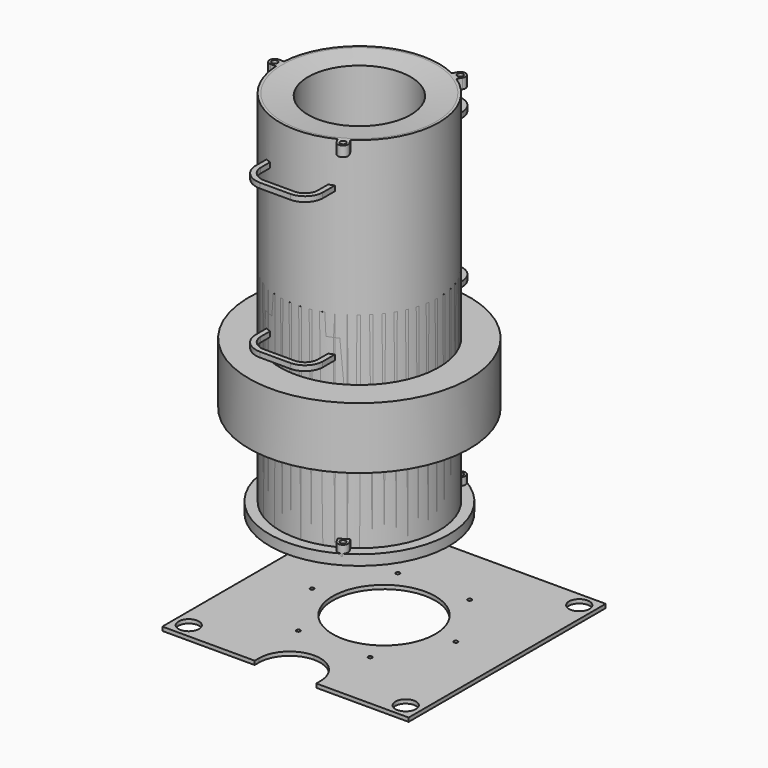
from build123d import *

# Parameters (mm, degrees)
F0_R      = 25.4
F0_R_2    = 4.7625
F1_DEPTH  = 9.525
F2_R      = 3.175
F3_DEPTH  = 12.7
F7_START  = -488.95
F6_R      = 7.14375
F7_DEPTH  = 25.4
F8_START  = -88.9
F8_DEPTH  = 12.7
F4_W      = 6.35
F4_H      = 381
F10_START = 266.7
F10_DEPTH = 12.7
F11_START = 355.6
F11_DEPTH = 25.4


# Not quite as in the source:
# - a feature names something its author has since deleted; it is built from what else it names


with BuildPart() as f1:
    # F0 (on Top) → F1 (new body)
    with BuildSketch(Plane.XY):
        with BuildLine():
            Line((609.6, 0), (0, 0))
            Line((0, 0), (0, -609.6))
            Line((0, -609.6), (228.6, -609.6))
            Line((228.6, -609.6), (228.6, -596.9))
            ThreePointArc((228.6, -596.9), (250.9184632736, -543.0184632736), (304.8, -520.7))
            ThreePointArc((304.8, -520.7), (358.6815367264, -543.0184632736), (381, -596.9))
            Line((381, -596.9), (381, -609.6))
            Line((381, -609.6), (609.6, -609.6))
            Line((609.6, -609.6), (609.6, 0))
        make_face()
        with Locations((36.3869200975, -573.2130799025)):
            Circle(F0_R, mode=Mode.SUBTRACT)
        with Locations((215.9, -458.7793167929)):
            Circle(F0_R_2, mode=Mode.SUBTRACT)
        with BuildLine():
            ThreePointArc((398.4625, -458.7793167929), (391.31875, -462.9037627784), (391.31875, -454.6548708073))
            ThreePointArc((391.31875, -454.6548708073), (396.08125, -454.6548708073), (398.4625, -458.7793167929))
        make_face(mode=Mode.SUBTRACT)
        with Locations((573.2130799025, -573.2130799025)):
            Circle(F0_R, mode=Mode.SUBTRACT)
        with Locations((127, -304.8)):
            Circle(F0_R_2, mode=Mode.SUBTRACT)
        with Locations((36.3869200975, -36.3869200975)):
            Circle(F0_R, mode=Mode.SUBTRACT)
        with Locations((215.9, -150.8206832071)):
            Circle(F0_R_2, mode=Mode.SUBTRACT)
        with BuildLine():
            ThreePointArc((368.3, -414.7852262806), (337.670018728, -427.4725799387), (304.8, -431.8))
            ThreePointArc((304.8, -431.8), (214.9974387893, -214.9974387893), (431.8, -304.8))
            ThreePointArc((431.8, -304.8), (414.7852262806, -368.3), (368.3, -414.7852262806))
        make_face(mode=Mode.SUBTRACT)
        with Locations((482.6, -304.8)):
            Circle(F0_R_2, mode=Mode.SUBTRACT)
        with Locations((393.7, -150.8206832071)):
            Circle(F0_R_2, mode=Mode.SUBTRACT)
        with Locations((573.2130799025, -36.3869200975)):
            Circle(F0_R, mode=Mode.SUBTRACT)
    extrude(amount=-F1_DEPTH)


with BuildPart() as f3:
    # F2 (on Top) → F3 (new body)
    with BuildSketch(Plane.XY):
        with BuildLine():
            ThreePointArc((13.051756509, -139.0889702745), (103.2942892524, -94.0551955388), (139.7, 0))
            ThreePointArc((139.7, 0), (93.8175544432, 103.5101757234), (-13.6909302547, 139.0275096115))
            Line((-13.6909302547, 139.0275096115), (-12.1714498273, 123.2253371732))
            ThreePointArc((-12.1714498273, 123.2253371732), (-9.8348553071, 122.5039217735), (-8.7041161086, 120.3356175983))
            ThreePointArc((-8.7041161086, 120.3356175983), (3.9055898005, 120.5867690433), (16.4726167188, 119.5201882463))
            ThreePointArc((16.4726167188, 119.5201882463), (19.8499978481, 122.2114111712), (22.7869087337, 119.0453507527))
            ThreePointArc((22.7869087337, 119.0453507527), (22.7745623185, 118.7656235596), (22.7376190943, 118.4880718804))
            ThreePointArc((22.7376190943, 118.4880718804), (34.982662471, 115.467033505), (46.8454269076, 111.1842096605))
            ThreePointArc((46.8454269076, 111.1842096606), (50.4041591942, 113.0209407678), (52.9298531544, 109.9130433005))
            ThreePointArc((52.9298531544, 109.9130433005), (52.853938074, 109.2229000827), (52.6298231316, 108.5657598745))
            ThreePointArc((52.6298231316, 108.5657598745), (63.6757245056, 102.4784104516), (74.0257986684, 95.271210927))
            ThreePointArc((74.0257986684, 95.271210927), (77.5564997152, 96.286901116), (79.6820865564, 93.2903435874))
            ThreePointArc((79.6820865564, 93.2903435874), (79.4895766086, 92.2015928865), (78.9353916974, 91.2448707467))
            ThreePointArc((78.9353916974, 91.2448707467), (88.0293911444, 82.5060530795), (96.1614345834, 72.8656366119))
            ThreePointArc((96.1614345834, 72.8656366119), (99.4770529713, 73.1440067882), (101.2204884435, 70.3100611283))
            ThreePointArc((101.2204884435, 70.3100611283), (100.8603523966, 68.8413317708), (99.8616437659, 67.7057944667))
            ThreePointArc((99.8616437659, 67.7057944667), (106.3840002521, 56.9110445377), (111.7438276458, 45.4943895779))
            ThreePointArc((111.7438276458, 45.4943895779), (114.6914737518, 45.1611083914), (116.0772523211, 42.5382641963))
            ThreePointArc((116.0772523211, 42.5382641963), (115.5013270724, 40.7146865486), (113.982489841, 39.5526801829))
            ThreePointArc((113.982489841, 39.552680183), (117.4887155504, 27.4376423606), (119.7110635196, 15.0227750771))
            ThreePointArc((119.7110635196, 15.0227750771), (122.1811785416, 14.2344199961), (123.2399142827, 11.867554857))
            ThreePointArc((123.2399142827, 11.867554857), (122.4037289426, 9.7203308383), (120.3356175983, 8.7041161086))
            ThreePointArc((120.3356175983, 8.7041161086), (120.5713787829, 4.3548959094), (120.65, 0))
            ThreePointArc((120.65, 0), (120.3672156609, -8.2556583045), (119.5201882463, -16.4726167188))
            ThreePointArc((119.5201882463, -16.4726167188), (121.4524479715, -17.5415203694), (122.2203507527, -19.6119087337))
            ThreePointArc((122.2203507527, -19.6119087337), (121.0838875539, -22.0460395251), (118.4880718804, -22.7376190943))
            ThreePointArc((118.4880718804, -22.7376190943), (115.467033505, -34.982662471), (111.1842096605, -46.8454269076))
            ThreePointArc((111.1842096606, -46.8454269076), (112.5697873786, -48.0163664839), (113.0880433005, -49.7548531544))
            ThreePointArc((113.0880433005, -49.7548531544), (111.6164223133, -52.4342420658), (108.5657598745, -52.6298231316))
            ThreePointArc((108.5657598745, -52.6298231316), (102.4784104516, -63.6757245056), (95.271210927, -74.0257986684))
            ThreePointArc((95.271210927, -74.0257986684), (96.1512768969, -75.1302475686), (96.4653435874, -76.5070865564))
            ThreePointArc((96.4653435874, -76.5070865564), (94.6294195245, -79.3858885007), (91.2448707467, -78.9353916974))
            ThreePointArc((91.2448707467, -78.9353916974), (82.5060530795, -88.0293911444), (72.8656366119, -96.1614345834))
            ThreePointArc((72.8656366119, -96.1614345834), (73.3262323072, -97.0538552352), (73.4850611283, -98.0454884435))
            ThreePointArc((73.4850611283, -98.0454884435), (71.2619220292, -101.0744463213), (67.7057944667, -99.8616437659))
            ThreePointArc((67.7057944667, -99.8616437659), (56.9110445377, -106.3840002521), (45.4943895779, -111.7438276458))
            ThreePointArc((45.4943895779, -111.7438276458), (45.6580657193, -112.3127920114), (45.7132641963, -112.9022523211))
            ThreePointArc((45.7132641963, -112.9022523211), (43.086623457, -116.0295398232), (39.5526801829, -113.982489841))
            ThreePointArc((39.552680183, -113.982489841), (27.4376423606, -117.4887155504), (15.0227750771, -119.7110635196))
            ThreePointArc((15.0227750771, -119.7110635196), (15.0376060553, -119.887712701), (15.042554857, -120.0649142827))
            ThreePointArc((15.042554857, -120.0649142827), (13.9884245204, -122.4276535555), (11.5259961981, -123.2214887999))
            Line((11.5259961981, -123.2214887999), (13.051756509, -139.0889702745))
        make_face()
        with BuildLine():
            Line((-12.1714498273, 123.2253371732), (-13.6909302547, 139.0275096115))
            ThreePointArc((-13.6909302547, 139.0275096115), (-139.0586071835, -13.3713786943), (13.051756509, -139.0889702745))
            Line((13.051756509, -139.0889702745), (11.5259961981, -123.2214887999))
            ThreePointArc((11.5259961981, -123.2214887999), (9.5974634812, -122.2846688064), (8.7041161086, -120.3356175983))
            ThreePointArc((8.7041161086, -120.3356175983), (-3.9055898005, -120.5867690433), (-16.4726167188, -119.5201882463))
            ThreePointArc((-16.4726167188, -119.5201882463), (-20.1280115951, -122.1781231409), (-22.7376190943, -118.4880718804))
            ThreePointArc((-22.7376190943, -118.4880718804), (-34.982662471, -115.467033505), (-46.8454269076, -111.1842096605))
            ThreePointArc((-46.8454269076, -111.1842096606), (-51.0641913953, -112.8054918085), (-52.6298231316, -108.5657598745))
            ThreePointArc((-52.6298231316, -108.5657598745), (-63.6757245056, -102.4784104516), (-74.0257986684, -95.271210927))
            ThreePointArc((-74.0257986684, -95.271210927), (-78.5204309394, -95.7453526292), (-78.9353916974, -91.2448707467))
            ThreePointArc((-78.9353916974, -91.2448707467), (-88.0293911444, -82.5060530795), (-96.1614345834, -72.8656366119))
            ThreePointArc((-96.1614345834, -72.8656366119), (-100.6256328762, -72.1603258949), (-99.8616437659, -67.7057944667))
            ThreePointArc((-99.8616437659, -67.7057944667), (-106.3840002521, -56.9110445377), (-111.7438276458, -45.4943895779))
            ThreePointArc((-111.7438276458, -45.4943895779), (-115.8733642242, -43.6576922014), (-113.982489841, -39.5526801829))
            ThreePointArc((-113.982489841, -39.552680183), (-117.4887155504, -27.4376423606), (-119.7110635196, -15.0227750771))
            ThreePointArc((-119.7110635196, -15.0227750771), (-123.2245172902, -12.1798589322), (-120.3356175983, -8.7041161086))
            ThreePointArc((-120.3356175983, -8.7041161086), (-120.5867690433, 3.9055898005), (-119.5201882463, 16.4726167188))
            ThreePointArc((-119.5201882463, 16.4726167188), (-122.1781231409, 20.1280115951), (-118.4880718804, 22.7376190943))
            ThreePointArc((-118.4880718804, 22.7376190943), (-115.467033505, 34.982662471), (-111.1842096605, 46.8454269076))
            ThreePointArc((-111.1842096606, 46.8454269076), (-112.8054918085, 51.0641913953), (-108.5657598745, 52.6298231316))
            ThreePointArc((-108.5657598745, 52.6298231316), (-102.4784104516, 63.6757245056), (-95.271210927, 74.0257986684))
            ThreePointArc((-95.271210927, 74.0257986684), (-95.7453526292, 78.5204309394), (-91.2448707467, 78.9353916974))
            ThreePointArc((-91.2448707467, 78.9353916974), (-82.5060530795, 88.0293911444), (-72.8656366119, 96.1614345834))
            ThreePointArc((-72.8656366119, 96.1614345834), (-72.1603258949, 100.6256328762), (-67.7057944667, 99.8616437659))
            ThreePointArc((-67.7057944667, 99.8616437659), (-56.9110445377, 106.3840002521), (-45.4943895779, 111.7438276458))
            ThreePointArc((-45.4943895779, 111.7438276458), (-43.6576922014, 115.8733642242), (-39.5526801829, 113.982489841))
            ThreePointArc((-39.552680183, 113.982489841), (-27.4376423606, 117.4887155504), (-15.0227750771, 119.7110635196))
            ThreePointArc((-15.0227750771, 119.7110635196), (-14.3330972524, 122.0653456603), (-12.1714498273, 123.2253371732))
        make_face()
        with BuildLine():
            ThreePointArc((-11.5636598867, 116.9044913922), (-13.8679862346, 117.5993718873), (-15.0227750771, 119.7110635196))
            ThreePointArc((-15.0227750771, 119.7110635196), (-27.4376423606, 117.4887155504), (-39.552680183, 113.982489841))
            ThreePointArc((-39.5526801829, 113.982489841), (-39.4109766941, 113.4506115818), (-39.3632641963, 112.9022523211))
            ThreePointArc((-39.3632641963, 112.9022523211), (-41.9488038866, 109.782450798), (-45.4943895779, 111.7438276458))
            ThreePointArc((-45.4943895779, 111.7438276458), (-56.9110445377, 106.3840002521), (-67.7057944667, 99.8616437659))
            ThreePointArc((-67.7057944667, 99.8616437659), (-67.2811032506, 98.9973493444), (-67.1350611283, 98.0454884435))
            ThreePointArc((-67.1350611283, 98.0454884435), (-69.31842792, 95.0293172647), (-72.8656366119, 96.1614345834))
            ThreePointArc((-72.8656366119, 96.1614345834), (-82.5060530795, 88.0293911444), (-91.2448707467, 78.9353916974))
            ThreePointArc((-91.2448707467, 78.9353916974), (-90.4115416431, 77.8461624935), (-90.1153435874, 76.5070865564))
            ThreePointArc((-90.1153435874, 76.5070865564), (-91.9135045996, 73.6461532468), (-95.271210927, 74.0257986684))
            ThreePointArc((-95.271210927, 74.0257986684), (-102.4784104516, 63.6757245056), (-108.5657598745, 52.6298231316))
            ThreePointArc((-108.5657598745, 52.6298231316), (-107.2336543891, 51.4582321672), (-106.7380433005, 49.7548531544))
            ThreePointArc((-106.7380433005, 49.7548531544), (-108.17455663, 47.0981090763), (-111.1842096606, 46.8454269076))
            ThreePointArc((-111.1842096605, 46.8454269076), (-115.467033505, 34.982662471), (-118.4880718804, 22.7376190943))
            ThreePointArc((-118.4880718804, 22.7376190943), (-116.6112199612, 21.650445535), (-115.8703507527, 19.6119087337))
            ThreePointArc((-115.8703507527, 19.6119087337), (-116.9749623884, 17.2048115148), (-119.5201882463, 16.4726167188))
            ThreePointArc((-119.5201882463, 16.4726167188), (-120.5867690433, 3.9055898005), (-120.3356175983, -8.7041161086))
            ThreePointArc((-120.3356175983, -8.7041161086), (-117.917690264, -9.5287401971), (-116.8899142827, -11.867554857))
            ThreePointArc((-116.8899142827, -11.867554857), (-117.6980491436, -13.9838191159), (-119.7110635196, -15.0227750771))
            ThreePointArc((-119.7110635196, -15.0227750771), (-117.4887155504, -27.4376423606), (-113.982489841, -39.552680183))
            ThreePointArc((-113.982489841, -39.5526801829), (-111.0786746734, -39.939189445), (-109.7272523211, -42.5382641963))
            ThreePointArc((-109.7272523211, -42.5382641963), (-110.2794081259, -44.327485627), (-111.7438276458, -45.4943895779))
            ThreePointArc((-111.7438276458, -45.4943895779), (-106.3840002521, -56.9110445377), (-99.8616437659, -67.7057944667))
            ThreePointArc((-99.8616437659, -67.7057944667), (-96.576759086, -67.4951971753), (-94.8704884435, -70.3100611283))
            ThreePointArc((-94.8704884435, -70.3100611283), (-95.2115427837, -71.7416256561), (-96.1614345834, -72.8656366119))
            ThreePointArc((-96.1614345834, -72.8656366119), (-88.0293911444, -82.5060530795), (-78.9353916974, -91.2448707467))
            ThreePointArc((-78.9353916974, -91.2448707467), (-75.4183358555, -90.3078535352), (-73.3320865564, -93.2903435874))
            ThreePointArc((-73.3320865564, -93.2903435874), (-73.5105290278, -94.3397567462), (-74.0257986684, -95.271210927))
            ThreePointArc((-74.0257986684, -95.271210927), (-63.6757245056, -102.4784104516), (-52.6298231316, -108.5657598745))
            ThreePointArc((-52.6298231316, -108.5657598745), (-49.0647099365, -106.8139583809), (-46.5798531544, -109.9130433005))
            ThreePointArc((-46.5798531544, -109.9130433005), (-46.6469556872, -110.5623493403), (-46.8454269076, -111.1842096606))
            ThreePointArc((-46.8454269076, -111.1842096605), (-34.982662471, -115.467033505), (-22.7376190943, -118.4880718804))
            ThreePointArc((-22.7376190943, -118.4880718804), (-19.3321815406, -115.8826971678), (-16.4369087337, -119.0453507527))
            ThreePointArc((-16.4369087337, -119.0453507527), (-16.4458483152, -119.2834398671), (-16.4726167188, -119.5201882463))
            ThreePointArc((-16.4726167188, -119.5201882463), (-3.9055898005, -120.5867690433), (8.7041161086, -120.3356175983))
            ThreePointArc((8.7041161086, -120.3356175983), (9.2345604525, -118.2906636055), (10.9307660245, -117.0312610917))
            Line((10.9307660245, -117.0312610917), (9.7026187096, -104.2588717264))
            ThreePointArc((9.7026187096, -104.2588717264), (6.883754478, -101.4061921796), (9.107388536, -98.0686440183))
            Line((9.107388536, -98.0686440183), (7.2714427619, -78.9753202821))
            ThreePointArc((7.2714427619, -78.9753202821), (4.4525785303, -76.1226407353), (6.6762125883, -72.7850925739))
            Line((6.6762125883, -72.7850925739), (4.8402506288, -53.6916005141))
            ThreePointArc((4.8402506288, -53.6916005141), (2.0213863972, -50.8389209672), (4.2450204553, -47.5013728059))
            Line((4.2450204553, -47.5013728059), (2.4089937501, -28.4072074092))
            ThreePointArc((2.4089937501, -28.4072074092), (-0.4098704815, -25.5545278623), (1.8137635765, -22.216979701))
            Line((1.8137635765, -22.216979701), (-0.0172496444, -3.1749531414))
            ThreePointArc((-0.0172496444, -3.1749531414), (-3.1604228905, -0.3038949703), (-0.6219241013, 3.1134924783))
            Line((-0.6219241013, 3.1134924783), (-2.4466574387, 22.0902100014))
            ThreePointArc((-2.4466574387, 22.0902100014), (-5.9109752996, 24.9467379216), (-3.0544473793, 28.4110557825))
            Line((-3.0544473793, 28.4110557825), (-4.8779143174, 47.3746031063))
            ThreePointArc((-4.8779143174, 47.3746031063), (-8.3422321783, 50.2311310266), (-5.4857042581, 53.6954488874))
            Line((-5.4857042581, 53.6954488874), (-7.3091064505, 72.6583228744))
            ThreePointArc((-7.3091064505, 72.6583228744), (-10.7734243114, 75.5148507946), (-7.9168963912, 78.9791686555))
            Line((-7.9168963912, 78.9791686555), (-9.7402823982, 97.9418743187))
            ThreePointArc((-9.7402823982, 97.9418743187), (-13.204600259, 100.7984022389), (-10.3480723388, 104.2627200998))
            Line((-10.3480723388, 104.2627200998), (-11.5636598867, 116.9044913922))
        make_face()
        with Locations((-41.8526358434, -92.5792464484)):
            Circle(F2_R, mode=Mode.SUBTRACT)
        with Locations((-12.2697406918, -75.2056744093)):
            Circle(F2_R, mode=Mode.SUBTRACT)
        with Locations((-82.5350690799, -59.2496613659)):
            Circle(F2_R, mode=Mode.SUBTRACT)
        with Locations((-71.2648948931, -26.9769300677)):
            Circle(F2_R, mode=Mode.SUBTRACT)
        with Locations((-101.1022972093, -10.0441773685)):
            Circle(F2_R, mode=Mode.SUBTRACT)
        with Locations((-75.8187457649, -7.6130014208)):
            Circle(F2_R, mode=Mode.SUBTRACT)
        with Locations((-48.2287443416, -58.9951542013)):
            Circle(F2_R, mode=Mode.SUBTRACT)
        with Locations((-61.8544592051, -44.5024255119)):
            Circle(F2_R, mode=Mode.SUBTRACT)
        with Locations((-31.316320253, -69.4674606259)):
            Circle(F2_R, mode=Mode.SUBTRACT)
        with Locations((-20.7799345177, -46.3555209381)):
            Circle(F2_R, mode=Mode.SUBTRACT)
        with Locations((-41.1737116503, -29.7550914792)):
            Circle(F2_R, mode=Mode.SUBTRACT)
        with Locations((-50.5350259969, -5.1818092878)):
            Circle(F2_R, mode=Mode.SUBTRACT)
        with Locations((-10.2432681853, -23.2429657506)):
            Circle(F2_R, mode=Mode.SUBTRACT)
        with Locations((-20.4924133416, -15.0073647066)):
            Circle(F2_R, mode=Mode.SUBTRACT)
        with Locations((-25.250632892, -2.750552409)):
            Circle(F2_R, mode=Mode.SUBTRACT)
        with Locations((-75.2056744093, 12.2697406918)):
            Circle(F2_R, mode=Mode.SUBTRACT)
        with Locations((-92.5792464484, 41.8526358434)):
            Circle(F2_R, mode=Mode.SUBTRACT)
        with Locations((-69.4674606259, 31.316320253)):
            Circle(F2_R, mode=Mode.SUBTRACT)
        with Locations((-46.3555209381, 20.7799345177)):
            Circle(F2_R, mode=Mode.SUBTRACT)
        with Locations((-23.2429657506, 10.2432681853)):
            Circle(F2_R, mode=Mode.SUBTRACT)
        with Locations((-15.0073647066, 20.4924133416)):
            Circle(F2_R, mode=Mode.SUBTRACT)
        with Locations((-58.9951542013, 48.2287443416)):
            Circle(F2_R, mode=Mode.SUBTRACT)
        with Locations((-44.5024255119, 61.8544592051)):
            Circle(F2_R, mode=Mode.SUBTRACT)
        with Locations((-29.7550914792, 41.1737116503)):
            Circle(F2_R, mode=Mode.SUBTRACT)
        with Locations((-59.2496613659, 82.5350690799)):
            Circle(F2_R, mode=Mode.SUBTRACT)
        with Locations((-26.9769300677, 71.2648948931)):
            Circle(F2_R, mode=Mode.SUBTRACT)
        with BuildLine():
            ThreePointArc((16.4726167188, 119.5201882463), (3.9055898005, 120.5867690433), (-8.7041161086, 120.3356175983))
            ThreePointArc((-8.7041161086, 120.3356175983), (-8.6954464867, 120.2003893243), (-8.692554857, 120.0649142827))
            ThreePointArc((-8.692554857, 120.0649142827), (-9.5175025671, 117.9299952598), (-11.5636598867, 116.9044913922))
            Line((-11.5636598867, 116.9044913922), (-10.3480723388, 104.2627200998))
            ThreePointArc((-10.3480723388, 104.2627200998), (-7.9092583455, 103.4523494992), (-6.8691773685, 101.1022972093))
            ThreePointArc((-6.8691773685, 101.1022972093), (-7.6941250786, 98.9673781863), (-9.7402823982, 97.9418743187))
            Line((-9.7402823982, 97.9418743187), (-7.9168963912, 78.9791686555))
            ThreePointArc((-7.9168963912, 78.9791686555), (-5.4780823979, 78.1687980549), (-4.4380014208, 75.8187457649))
            ThreePointArc((-4.4380014208, 75.8187457649), (-5.2629491309, 73.683826742), (-7.3091064505, 72.6583228744))
            Line((-7.3091064505, 72.6583228744), (-5.4857042581, 53.6954488874))
            ThreePointArc((-5.4857042581, 53.6954488874), (-3.0468902648, 52.8850782868), (-2.0068092878, 50.5350259969))
            ThreePointArc((-2.0068092878, 50.5350259969), (-2.8317569978, 48.4001069739), (-4.8779143174, 47.3746031063))
            Line((-4.8779143174, 47.3746031063), (-3.0544473793, 28.4110557825))
            ThreePointArc((-3.0544473793, 28.4110557825), (-0.6156333861, 27.6006851819), (0.424447591, 25.250632892))
            ThreePointArc((0.424447591, 25.250632892), (-0.4005001191, 23.115713869), (-2.4466574387, 22.0902100014))
            Line((-2.4466574387, 22.0902100014), (-0.6219241013, 3.1134924783))
            ThreePointArc((-0.6219241013, 3.1134924783), (2.013208382, 2.4551205695), (3.175, 0))
            ThreePointArc((3.175, 0), (2.238957054, -2.2511544395), (-0.0172496444, -3.1749531414))
            Line((-0.0172496444, -3.1749531414), (1.8137635765, -22.216979701))
            ThreePointArc((1.8137635765, -22.216979701), (4.6355352282, -22.6957425281), (5.925552409, -25.250632892))
            ThreePointArc((5.925552409, -25.250632892), (4.8714220724, -27.6133721647), (2.4089937501, -28.4072074092))
            Line((2.4089937501, -28.4072074092), (4.2450204553, -47.5013728059))
            ThreePointArc((4.2450204553, -47.5013728059), (7.0667921069, -47.980135633), (8.3568092878, -50.5350259969))
            ThreePointArc((8.3568092878, -50.5350259969), (7.3026789511, -52.8977652696), (4.8402506288, -53.6916005141))
            Line((4.8402506288, -53.6916005141), (6.6762125883, -72.7850925739))
            ThreePointArc((6.6762125883, -72.7850925739), (9.49798424, -73.263855401), (10.7880014208, -75.8187457649))
            ThreePointArc((10.7880014208, -75.8187457649), (9.7338710842, -78.1814850377), (7.2714427619, -78.9753202821))
            Line((7.2714427619, -78.9753202821), (9.107388536, -98.0686440183))
            ThreePointArc((9.107388536, -98.0686440183), (11.9291601876, -98.5474068454), (13.2191773685, -101.1022972093))
            ThreePointArc((13.2191773685, -101.1022972093), (12.1650470319, -103.465036482), (9.7026187096, -104.2588717264))
            Line((9.7026187096, -104.2588717264), (10.9307660245, -117.0312610917))
            ThreePointArc((10.9307660245, -117.0312610917), (13.6070072762, -117.4088024098), (15.0227750771, -119.7110635196))
            ThreePointArc((15.0227750771, -119.7110635196), (27.4376423606, -117.4887155504), (39.552680183, -113.982489841))
            ThreePointArc((39.5526801829, -113.982489841), (41.4188361911, -109.9311404179), (45.4943895779, -111.7438276458))
            ThreePointArc((45.4943895779, -111.7438276458), (56.9110445377, -106.3840002521), (67.7057944667, -99.8616437659))
            ThreePointArc((67.7057944667, -99.8616437659), (68.4597963618, -95.4653440108), (72.8656366119, -96.1614345834))
            ThreePointArc((72.8656366119, -96.1614345834), (82.5060530795, -88.0293911444), (91.2448707467, -78.9353916974))
            ThreePointArc((91.2448707467, -78.9353916974), (90.8353345456, -74.4937421733), (95.271210927, -74.0257986684))
            ThreePointArc((95.271210927, -74.0257986684), (102.4784104516, -63.6757245056), (108.5657598745, -52.6298231316))
            ThreePointArc((108.5657598745, -52.6298231316), (107.0205947926, -48.4455149135), (111.1842096606, -46.8454269076))
            ThreePointArc((111.1842096605, -46.8454269076), (115.467033505, -34.982662471), (118.4880718804, -22.7376190943))
            ThreePointArc((118.4880718804, -22.7376190943), (115.9125783644, -19.0958058723), (119.5201882463, -16.4726167188))
            ThreePointArc((119.5201882463, -16.4726167188), (120.3672156609, -8.2556583045), (120.65, 0))
            ThreePointArc((120.65, 0), (120.5713787829, 4.3548959094), (120.3356175983, 8.7041161086))
            ThreePointArc((120.3356175983, 8.7041161086), (116.9053112753, 11.5552507818), (119.7110635196, 15.0227750771))
            ThreePointArc((119.7110635196, 15.0227750771), (117.4887155504, 27.4376423606), (113.982489841, 39.552680183))
            ThreePointArc((113.982489841, 39.5526801829), (109.9311404179, 41.4188361911), (111.7438276458, 45.4943895779))
            ThreePointArc((111.7438276458, 45.4943895779), (106.3840002521, 56.9110445377), (99.8616437659, 67.7057944667))
            ThreePointArc((99.8616437659, 67.7057944667), (95.4653440108, 68.4597963618), (96.1614345834, 72.8656366119))
            ThreePointArc((96.1614345834, 72.8656366119), (88.0293911444, 82.5060530795), (78.9353916974, 91.2448707467))
            ThreePointArc((78.9353916974, 91.2448707467), (74.4937421733, 90.8353345456), (74.0257986684, 95.271210927))
            ThreePointArc((74.0257986684, 95.271210927), (63.6757245056, 102.4784104516), (52.6298231316, 108.5657598745))
            ThreePointArc((52.6298231316, 108.5657598745), (48.4455149135, 107.0205947926), (46.8454269076, 111.1842096606))
            ThreePointArc((46.8454269076, 111.1842096605), (34.982662471, 115.467033505), (22.7376190943, 118.4880718804))
            ThreePointArc((22.7376190943, 118.4880718804), (19.0958058723, 115.9125783644), (16.4726167188, 119.5201882463))
        make_face()
        with Locations((26.9769300677, -71.2648948931)):
            Circle(F2_R, mode=Mode.SUBTRACT)
        with Locations((59.2496613659, -82.5350690799)):
            Circle(F2_R, mode=Mode.SUBTRACT)
        with Locations((29.7550914792, -41.1737116503)):
            Circle(F2_R, mode=Mode.SUBTRACT)
        with Locations((44.5024255119, -61.8544592051)):
            Circle(F2_R, mode=Mode.SUBTRACT)
        with Locations((58.9951542013, -48.2287443416)):
            Circle(F2_R, mode=Mode.SUBTRACT)
        with Locations((15.0073647066, -20.4924133416)):
            Circle(F2_R, mode=Mode.SUBTRACT)
        with Locations((23.2429657506, -10.2432681853)):
            Circle(F2_R, mode=Mode.SUBTRACT)
        with Locations((46.3555209381, -20.7799345177)):
            Circle(F2_R, mode=Mode.SUBTRACT)
        with Locations((69.4674606259, -31.316320253)):
            Circle(F2_R, mode=Mode.SUBTRACT)
        with Locations((92.5792464484, -41.8526358434)):
            Circle(F2_R, mode=Mode.SUBTRACT)
        with Locations((75.2056744093, -12.2697406918)):
            Circle(F2_R, mode=Mode.SUBTRACT)
        with Locations((25.250632892, 2.750552409)):
            Circle(F2_R, mode=Mode.SUBTRACT)
        with Locations((20.4924133416, 15.0073647066)):
            Circle(F2_R, mode=Mode.SUBTRACT)
        with Locations((10.2432681853, 23.2429657506)):
            Circle(F2_R, mode=Mode.SUBTRACT)
        with Locations((50.5350259969, 5.1818092878)):
            Circle(F2_R, mode=Mode.SUBTRACT)
        with Locations((41.1737116503, 29.7550914792)):
            Circle(F2_R, mode=Mode.SUBTRACT)
        with Locations((20.7799345177, 46.3555209381)):
            Circle(F2_R, mode=Mode.SUBTRACT)
        with Locations((31.316320253, 69.4674606259)):
            Circle(F2_R, mode=Mode.SUBTRACT)
        with Locations((61.8544592051, 44.5024255119)):
            Circle(F2_R, mode=Mode.SUBTRACT)
        with Locations((48.2287443416, 58.9951542013)):
            Circle(F2_R, mode=Mode.SUBTRACT)
        with Locations((75.8187457649, 7.6130014208)):
            Circle(F2_R, mode=Mode.SUBTRACT)
        with Locations((101.1022972093, 10.0441773685)):
            Circle(F2_R, mode=Mode.SUBTRACT)
        with Locations((71.2648948931, 26.9769300677)):
            Circle(F2_R, mode=Mode.SUBTRACT)
        with Locations((82.5350690799, 59.2496613659)):
            Circle(F2_R, mode=Mode.SUBTRACT)
        with Locations((12.2697406918, 75.2056744093)):
            Circle(F2_R, mode=Mode.SUBTRACT)
        with Locations((41.8526358434, 92.5792464484)):
            Circle(F2_R, mode=Mode.SUBTRACT)
    extrude(amount=F3_DEPTH)


with BuildPart() as f5:
    # F4 (on Right) → F5 (revolve)
    with BuildSketch(Plane.YZ):
        with BuildLine():
            Line((127, 533.4), (127, 0))
            ThreePointArc((127, 0), (159.9015290315, 4.3910069739), (190.5, 17.2566639429))
            Line((190.5, 17.2566639429), (190.5, 533.4))
            Line((190.5, 533.4), (127, 533.4))
        make_face()
        Polygon((190.5, 533.4), (190.5, 17.2566639429), (196.85, 18.9823303372), (196.85, 25.4), (196.85, 228.6), (196.85, 234.9500060081), (196.85, 374.6500015259), (196.85, 381), (196.85, 533.4), align=None)
    revolve(axis=Axis((0, 0, 69.85), (0, 0, 1)))

    # F6 (on face) → F7 (join)
    with BuildSketch(Plane.XY.offset(533.4).offset(F7_START)):
        with BuildLine():
            ThreePointArc((109.1282377053, -163.8320793841), (98.425, -170.477100735), (87.3186238488, -176.4238658151))
            Line((87.3186238488, -176.4238658151), (93.8160862872, -187.6778008787))
            ThreePointArc((93.8160862872, -187.6778008787), (111.016786431, -192.2867145915), (115.6257001437, -175.0860144477))
            Line((115.6257001437, -175.0860144477), (109.1282377053, -163.8320793841))
        make_face()
        with Locations((104.7208932155, -181.3819076632)):
            Circle(F6_R, mode=Mode.SUBTRACT)
        with BuildLine():
            Line((-196.4468615542, 12.591786431), (-209.441786431, 12.591786431))
            ThreePointArc((-209.441786431, 12.591786431), (-218.3455240036, 8.9037375726), (-222.0335728619, 0))
            Line((-222.0335728619, 0), (-216.585536431, 0))
            ThreePointArc((-216.585536431, 0), (-209.441786431, 7.14375), (-202.298036431, 0))
            Line((-202.298036431, 0), (-196.85, 0))
            ThreePointArc((-196.85, 0), (-196.7491895751, 6.2991191077), (-196.4468615542, 12.591786431))
        make_face()
        with BuildLine():
            Line((-216.585536431, 0), (-222.0335728619, 0))
            ThreePointArc((-222.0335728619, 0), (-218.3455240036, -8.9037375726), (-209.441786431, -12.591786431))
            Line((-209.441786431, -12.591786431), (-196.4468615542, -12.591786431))
            ThreePointArc((-196.4468615542, -12.591786431), (-196.7491895751, -6.2991191077), (-196.85, 0))
            Line((-196.85, 0), (-202.298036431, 0))
            ThreePointArc((-202.298036431, 0), (-209.441786431, -7.14375), (-216.585536431, 0))
        make_face()
        with BuildLine():
            Line((93.8160862872, 187.6778008787), (87.3186238488, 176.4238658151))
            ThreePointArc((87.3186238488, 176.4238658151), (98.425, 170.477100735), (109.1282377053, 163.8320793841))
            Line((109.1282377053, 163.8320793841), (115.6257001437, 175.0860144477))
            ThreePointArc((115.6257001437, 175.0860144477), (111.016786431, 192.2867145915), (93.8160862872, 187.6778008787))
        make_face()
        with Locations((104.7208932155, 181.3819076632)):
            Circle(F6_R, mode=Mode.SUBTRACT)
    extrude(amount=-F7_DEPTH)

    # F6 (on face) → F8 (join)
    with BuildSketch(Plane.XY.offset(533.4).offset(F8_START)):
        with BuildLine():
            Line((-88.7907175359, 211.2049731988), (-88.7907175359, 175.6875948366))
            ThreePointArc((-88.7907175359, 175.6875948366), (-82.4927973706, 178.7312532322), (-76.0907175359, 181.5492363103))
            Line((-76.0907175359, 181.5492363103), (-76.0907175359, 210.891750467))
            ThreePointArc((-76.0907175359, 210.891750467), (-64.2969439267, 236.7542896981), (-38.0434198121, 247.65))
            Line((-38.0434198121, 247.65), (38.0422199188, 247.65))
            ThreePointArc((38.0422199188, 247.65), (59.9778029813, 238.5458979623), (69.85, 216.9451062124))
            Line((69.85, 216.9451062124), (69.85, 184.0404846766))
            ThreePointArc((69.85, 184.0404846766), (76.2466869761, 181.483787775), (82.55, 178.7048404493))
            Line((82.55, 178.7048404493), (82.55, 217.2617539162))
            ThreePointArc((82.55, 217.2617539162), (68.8853928159, 247.598821046), (38.1532180341, 260.35))
            Line((38.1532180341, 260.35), (-38.1532180341, 260.35))
            ThreePointArc((-38.1532180341, 260.35), (-73.2053190264, 245.8064274855), (-88.7907175359, 211.2049731988))
        make_face()
        with BuildLine():
            ThreePointArc((-76.0907175359, -181.5492363103), (-82.4927973706, -178.7312532322), (-88.7907175359, -175.6875948366))
            Line((-88.7907175359, -175.6875948366), (-88.7907175359, -211.2049731988))
            ThreePointArc((-88.7907175359, -211.2049731988), (-73.2053190264, -245.8064274855), (-38.1532180341, -260.35))
            Line((-38.1532180341, -260.35), (38.1532180341, -260.35))
            ThreePointArc((38.1532180341, -260.35), (68.8853928159, -247.598821046), (82.55, -217.2617539162))
            Line((82.55, -217.2617539162), (82.55, -178.7048404493))
            ThreePointArc((82.55, -178.7048404493), (76.2466869761, -181.483787775), (69.85, -184.0404846766))
            Line((69.85, -184.0404846766), (69.85, -216.9451062124))
            ThreePointArc((69.85, -216.9451062124), (59.9778029813, -238.5458979623), (38.0422199188, -247.65))
            Line((38.0422199188, -247.65), (-38.0434198121, -247.65))
            ThreePointArc((-38.0434198121, -247.65), (-64.2969439267, -236.7542896981), (-76.0907175359, -210.891750467))
            Line((-76.0907175359, -210.891750467), (-76.0907175359, -181.5492363103))
        make_face()
    extrude(amount=-F8_DEPTH)


with BuildPart() as f9:
    # F4 (on Right) → F9 (revolve)
    with BuildSketch(Plane.YZ):
        with BuildLine():
            Line((127, 533.4), (127, 0))
            ThreePointArc((127, 0), (159.9015290315, 4.3910069739), (190.5, 17.2566639429))
            Line((190.5, 17.2566639429), (190.5, 533.4))
            Line((190.5, 533.4), (127, 533.4))
        make_face()
        Polygon((190.5, 533.4), (190.5, 17.2566639429), (196.85, 18.9823303372), (196.85, 25.4), (196.85, 228.6), (196.85, 234.9500060081), (196.85, 374.6500015259), (196.85, 381), (196.85, 533.4), align=None)
        Polygon((127, 908.4164500237), (127, 533.4), (190.5, 533.4), (190.5, 914.4), align=None)
        with Locations((193.675, 723.9)):
            Rectangle(F4_W, F4_H)
        with BuildLine():
            ThreePointArc((190.5, 17.2566639429), (159.9015290315, 4.3910069739), (127, 0))
            Line((127, 0), (196.85, 0))
            Line((196.85, 0), (196.85, 18.9823303372))
            Line((196.85, 18.9823303372), (190.5, 17.2566639429))
        make_face()
        Polygon((196.85, 18.9823303372), (196.85, 0), (222.25, 0), (222.25, 25.4), (196.85, 25.4), align=None)
    revolve(axis=Axis((0, 0, 69.85), (0, 0, 1)))

    # F6 (on face) → F10 (join)
    with BuildSketch(Plane.XY.offset(533.4).offset(F10_START)):
        with BuildLine():
            Line((-88.7907175359, 211.2049731988), (-88.7907175359, 175.6875948366))
            ThreePointArc((-88.7907175359, 175.6875948366), (-82.4927973706, 178.7312532322), (-76.0907175359, 181.5492363103))
            Line((-76.0907175359, 181.5492363103), (-76.0907175359, 210.891750467))
            ThreePointArc((-76.0907175359, 210.891750467), (-64.2969439267, 236.7542896981), (-38.0434198121, 247.65))
            Line((-38.0434198121, 247.65), (38.0422199188, 247.65))
            ThreePointArc((38.0422199188, 247.65), (59.9778029813, 238.5458979623), (69.85, 216.9451062124))
            Line((69.85, 216.9451062124), (69.85, 184.0404846766))
            ThreePointArc((69.85, 184.0404846766), (76.2466869761, 181.483787775), (82.55, 178.7048404493))
            Line((82.55, 178.7048404493), (82.55, 217.2617539162))
            ThreePointArc((82.55, 217.2617539162), (68.8853928159, 247.598821046), (38.1532180341, 260.35))
            Line((38.1532180341, 260.35), (-38.1532180341, 260.35))
            ThreePointArc((-38.1532180341, 260.35), (-73.2053190264, 245.8064274855), (-88.7907175359, 211.2049731988))
        make_face()
        with BuildLine():
            ThreePointArc((-76.0907175359, -181.5492363103), (-82.4927973706, -178.7312532322), (-88.7907175359, -175.6875948366))
            Line((-88.7907175359, -175.6875948366), (-88.7907175359, -211.2049731988))
            ThreePointArc((-88.7907175359, -211.2049731988), (-73.2053190264, -245.8064274855), (-38.1532180341, -260.35))
            Line((-38.1532180341, -260.35), (38.1532180341, -260.35))
            ThreePointArc((38.1532180341, -260.35), (68.8853928159, -247.598821046), (82.55, -217.2617539162))
            Line((82.55, -217.2617539162), (82.55, -178.7048404493))
            ThreePointArc((82.55, -178.7048404493), (76.2466869761, -181.483787775), (69.85, -184.0404846766))
            Line((69.85, -184.0404846766), (69.85, -216.9451062124))
            ThreePointArc((69.85, -216.9451062124), (59.9778029813, -238.5458979623), (38.0422199188, -247.65))
            Line((38.0422199188, -247.65), (-38.0434198121, -247.65))
            ThreePointArc((-38.0434198121, -247.65), (-64.2969439267, -236.7542896981), (-76.0907175359, -210.891750467))
            Line((-76.0907175359, -210.891750467), (-76.0907175359, -181.5492363103))
        make_face()
    extrude(amount=F10_DEPTH)

    # F6 (on face) → F11 (join)
    with BuildSketch(Plane.XY.offset(533.4).offset(F11_START)):
        with BuildLine():
            Line((-216.585536431, 0), (-222.0335728619, 0))
            ThreePointArc((-222.0335728619, 0), (-218.3455240036, -8.9037375726), (-209.441786431, -12.591786431))
            Line((-209.441786431, -12.591786431), (-196.4468615542, -12.591786431))
            ThreePointArc((-196.4468615542, -12.591786431), (-196.7491895751, -6.2991191077), (-196.85, 0))
            Line((-196.85, 0), (-202.298036431, 0))
            ThreePointArc((-202.298036431, 0), (-209.441786431, -7.14375), (-216.585536431, 0))
        make_face()
        with BuildLine():
            Line((-196.4468615542, 12.591786431), (-209.441786431, 12.591786431))
            ThreePointArc((-209.441786431, 12.591786431), (-218.3455240036, 8.9037375726), (-222.0335728619, 0))
            Line((-222.0335728619, 0), (-216.585536431, 0))
            ThreePointArc((-216.585536431, 0), (-209.441786431, 7.14375), (-202.298036431, 0))
            Line((-202.298036431, 0), (-196.85, 0))
            ThreePointArc((-196.85, 0), (-196.7491895751, 6.2991191077), (-196.4468615542, 12.591786431))
        make_face()
        with BuildLine():
            Line((93.8160862872, 187.6778008787), (87.3186238488, 176.4238658151))
            ThreePointArc((87.3186238488, 176.4238658151), (98.425, 170.477100735), (109.1282377053, 163.8320793841))
            Line((109.1282377053, 163.8320793841), (115.6257001437, 175.0860144477))
            ThreePointArc((115.6257001437, 175.0860144477), (111.016786431, 192.2867145915), (93.8160862872, 187.6778008787))
        make_face()
        with Locations((104.7208932155, 181.3819076632)):
            Circle(F6_R, mode=Mode.SUBTRACT)
        with BuildLine():
            ThreePointArc((109.1282377053, -163.8320793841), (98.425, -170.477100735), (87.3186238488, -176.4238658151))
            Line((87.3186238488, -176.4238658151), (93.8160862872, -187.6778008787))
            ThreePointArc((93.8160862872, -187.6778008787), (111.016786431, -192.2867145915), (115.6257001437, -175.0860144477))
            Line((115.6257001437, -175.0860144477), (109.1282377053, -163.8320793841))
        make_face()
        with Locations((104.7208932155, -181.3819076632)):
            Circle(F6_R, mode=Mode.SUBTRACT)
    extrude(amount=F11_DEPTH)


with BuildPart() as f12:
    # F4 (on Right) → F12 (revolve)
    with BuildSketch(Plane.YZ):
        Polygon((273.05, 381), (196.85, 381), (196.85, 374.6500015259), (266.7000015259, 374.6500015259), (266.7000015259, 234.9500060081), (196.85, 234.9500060081), (196.85, 228.6), (273.05, 228.6), align=None)
    revolve(axis=Axis((0, 0, 69.85), (0, 0, 1)))


solid = Compound([f1.part, f3.part, f5.part, f9.part, f12.part])
